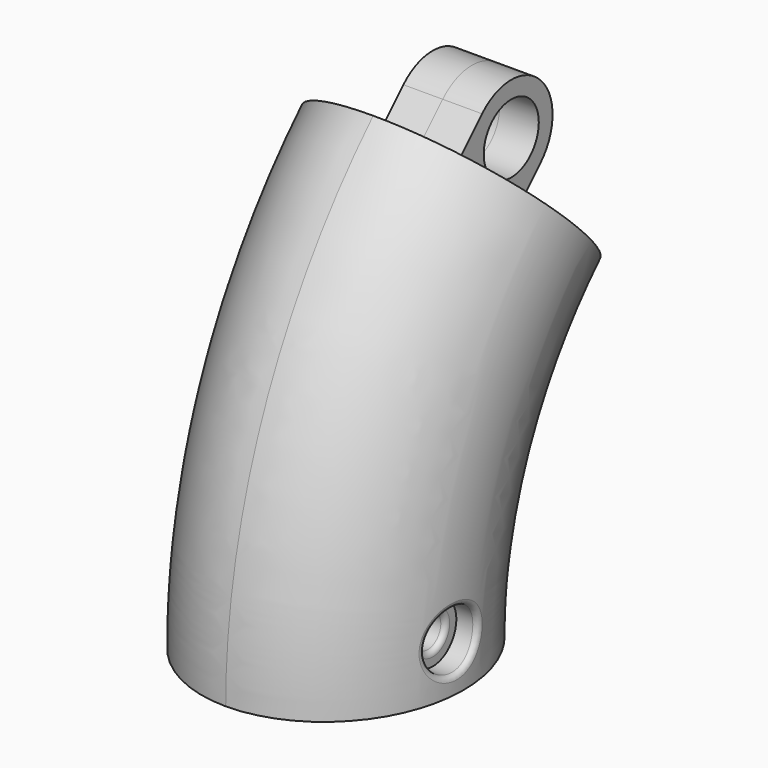
from build123d import *

# Parameters (mm, degrees)
F0_W      = 8.3
F0_H      = 10.8
F1_ANGLE  = 45
F3_DEPTH  = 10
F4_R      = 5.24999
F5_R      = 3.5
F6_DEPTH  = 17.0010001
F7_DEPTH  = 10.15
F8_R      = 5.39999
F9_W      = 20
F9_H      = 70
F10_DEPTH = 50
F11_R     = 3.35
F11_R_2   = 1.65
F12_DEPTH = 4.15
F13_DEPTH = 25
F14_R     = 3
F14_R_2   = 1.65
F15_DEPTH = 25
F16_DEPTH = 6.5
F17_R     = 0.5


# Not quite as in the source:
# - a fillet or chamfer is up to 0.001 mm smaller than in the source, because OpenCascade refuses the exact size
# - a feature names something its author has since deleted; it is built from what else it names


with BuildPart() as f1:
    # F0 (on Top) → F1 (revolve)
    with BuildSketch(Plane.XY):
        with BuildLine():
            add(Edge.make_bspline(
                [(0, 14), (-22.5166604984, 14), (-11.2583302492, -7), (0, -28), (11.2583302492, -7), (22.5166604984, 14), (0, 14)],
                knots=[0, 0, 0, 2.0943951024, 2.0943951024, 4.1887902048, 4.1887902048, 6.2831853072, 6.2831853072, 6.2831853072], degree=2, weights=[1, 0.5, 1, 0.5, 1, 0.5, 1]))
        make_face()
        with Locations((0, -1)):
            Rectangle(F0_W, F0_H, mode=Mode.SUBTRACT)
        with Locations((0, -1)):
            Rectangle(F0_W, F0_H)
    revolve(axis=Axis((13.7635422871, 50, 0), (-1, 0, 0)), revolution_arc=F1_ANGLE)

    # F2 (on face) → F3 (join)
    with BuildSketch(Plane(origin=(0, 25, 25), x_dir=(1, 0, 0), z_dir=(0, 0.7071067812, 0.7071067812))):
        Polygon((0, -10.3946609407), (-4, -10.3946609407), (-4, -20.8946609407), (4, -20.8946609407), (4, -10.3946609407), align=None)
    extrude(amount=F3_DEPTH)

    # F4 (radius 5.25 in the source; OpenCascade refuses exactly that, so slightly less here)
    f4_edges = [f1.edges().sort_by_distance(p)[0] for p in [
        (0, 17.296311, 46.845824),
        (0, 24.720933, 39.421203),
    ]]
    fillet(f4_edges, radius=F4_R)

    # F5 (on face) → F6 (cut, through all)
    with BuildSketch(Plane.YZ.offset(4)):
        with Locations((17.2963113701, 39.4212030512)):
            Circle(F5_R)
    extrude(amount=-F6_DEPTH, mode=Mode.SUBTRACT)

    # F0 (on Top) → F7 (cut)
    with BuildSketch(Plane.XY):
        with Locations((0, -1)):
            Rectangle(F0_W, F0_H)
    extrude(amount=F7_DEPTH, mode=Mode.SUBTRACT)

    # F8 (radius 5.4 in the source; OpenCascade refuses exactly that, so slightly less here)
    f8_edges = [f1.edges().sort_by_distance(p)[0] for p in [
        (0, 4.4, 10.15),
        (0, -6.4, 10.15),
    ]]
    fillet(f8_edges, radius=F8_R)

    # F9 (on Top) → F10 (intersect)
    with BuildSketch(Plane.XY):
        with Locations((10, 0)):
            Rectangle(F9_W, F9_H)
    extrude(amount=F10_DEPTH, mode=Mode.INTERSECT)

    # F11 (on face) → F12 (join)
    with BuildSketch(Plane(origin=(4.15, 0, 0), x_dir=(0, -1, 0), z_dir=(-1, 0, 0))):
        with Locations((1, 4.75)):
            Circle(F11_R)
        with Locations((1, 4.75)):
            Circle(F11_R_2, mode=Mode.SUBTRACT)
    extrude(amount=F12_DEPTH)

    # F13 (cut): a face of the model
    f13_faces = [f1.faces().sort_by_distance(p)[0] for p in [
        (4.15, -1, 4.75),
    ]]
    extrude(f13_faces, amount=-F13_DEPTH, mode=Mode.SUBTRACT)

    # F14 (on face) → F15 (cut)
    with BuildSketch(Plane(origin=(4.15, 0, 0), x_dir=(0, -1, 0), z_dir=(-1, 0, 0))):
        with Locations((1, 4.75)):
            Circle(F14_R)
        with Locations((1, 4.75)):
            Circle(F14_R_2, mode=Mode.SUBTRACT)
    extrude(amount=-F15_DEPTH, mode=Mode.SUBTRACT)

    # F14 (on face) → F16 (join)
    with BuildSketch(Plane(origin=(4.15, 0, 0), x_dir=(0, -1, 0), z_dir=(-1, 0, 0))):
        with Locations((1, 4.75)):
            Circle(F14_R)
        with Locations((1, 4.75)):
            Circle(F14_R_2, mode=Mode.SUBTRACT)
    extrude(amount=-F16_DEPTH)

    # F17
    f17_edges = [f1.edges().sort_by_distance(p)[0] for p in [
        (10.65, 0.65, 4.75),
        (12.896212, 2, 4.750084),
    ]]
    fillet(f17_edges, radius=F17_R)


with BuildPart() as f18_1:
    # F18: instance of F1
    add(f1.part.mirror(Plane.YZ))


solid = Compound([f1.part, f18_1.part])
